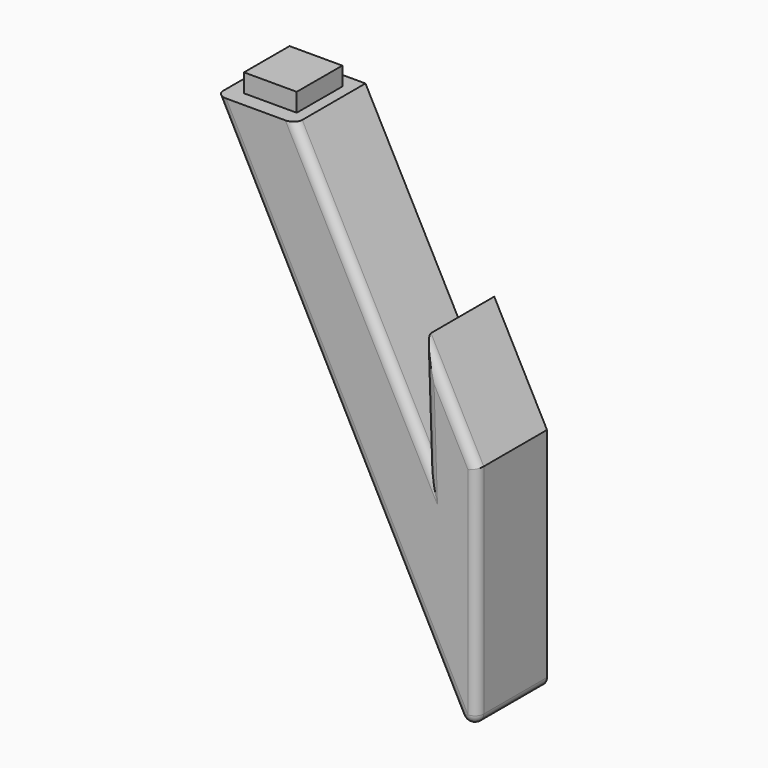
from build123d import *

# Parameters (mm, degrees)
F1_DEPTH = 10
F3_DEPTH = 2.1
F5_R     = 1


# Not quite as in the source:
# - a feature of the source that left no trace in its solid (it failed there, or was rolled back) is left out


with BuildPart() as f1:
    # F0 (on Front) → F1 (new body)
    with BuildSketch(Plane.XZ):
        Polygon((9, 0), (0, 0), (29.6767346319, -56.9180645261), (29.6767346319, -28.0180645261), (23.6665218482, -16.6037164372), (24.0578948756, -28.5973325372), align=None)
    extrude(amount=F1_DEPTH)

    # F2 (on face) → F3 (join)
    with BuildSketch(Plane.XY):
        Polygon((7.7660586685, -1.75), (1.75, -1.75), (1.75, -8.23), (7.75, -8.23), align=None)
    extrude(amount=F3_DEPTH)

    # F5
    f5_edges = [f1.edges().sort_by_distance(p)[0] for p in [
        (16.528947, -10, -14.298666),
        (23.862208, -10, -22.600524),
        (26.671628, -10, -22.31089),
        (29.676735, -10, -42.468065),
        (14.838367, -10, -28.459032),
        (29.676735, -5, -56.918065),
    ]]
    fillet(f5_edges, radius=F5_R)


solid = f1.part
